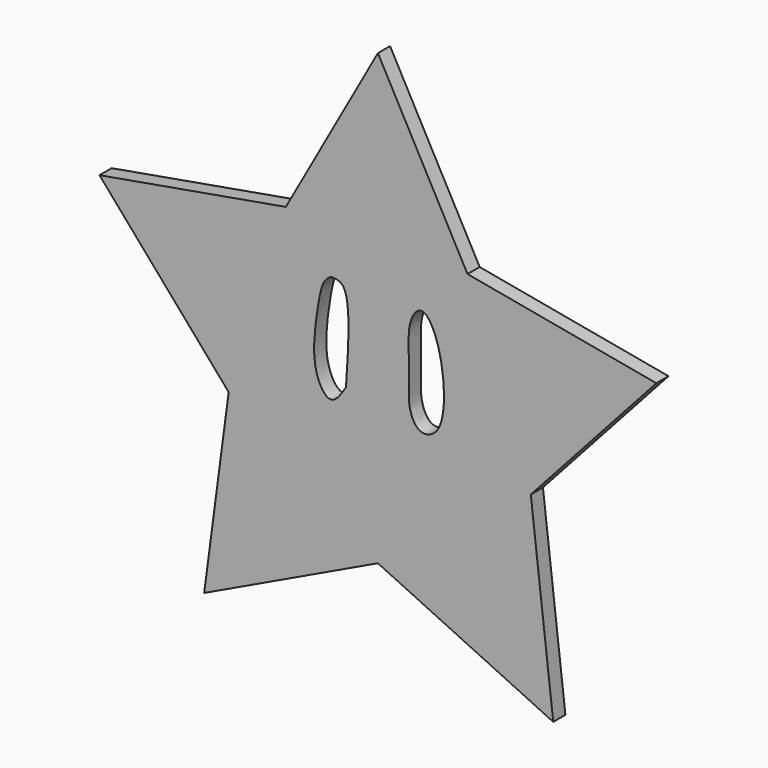
from build123d import *

# Parameters (mm, degrees)
F1_DEPTH = 2
F3_DEPTH = 25


with BuildPart() as f1:
    # F0 (on Front) → F1 (new body)
    with BuildSketch(Plane.XZ):
        Polygon((-48.7309247255, 48.1939427555), (-73.2373036639, 43.8981056213), (-56.2486425042, 24.2983382195), (-59.4705231488, 0), (-36.618651832, 10.8738420531), (-13.5587416589, 0), (-16.5121313184, 25.3722984344), (0, 43.6296164989), (-24.835318327, 48.1939427555), (-36.618651832, 69.941624999), align=None)
    extrude(amount=F1_DEPTH)

    # F2 (on face) → F3 (cut)
    with BuildSketch(Plane.XZ.offset(2)):
        with BuildLine():
            add(Edge.make_bspline(
                [(-42.8241454065, 42.018674314), (-42.215811031, 42.0156652147), (-40.0248783805, 42.0048278626), (-40.4838324873, 34.9711646084), (-40.8153533936, 29.8904683441)],
                knots=[0, 0, 0, 0, 0.2776600072, 1, 1, 1, 1], degree=3))
            add(Edge.make_bspline(
                [(-42.8241454065, 42.018674314), (-43.1211611971, 41.817411735), (-43.9730260473, 41.2401746918), (-44.7285981197, 37.046533313), (-45.4586501607, 30.6342959102), (-42.8138464069, 26.7380268066), (-41.4719755399, 28.85470644), (-40.8153533936, 29.8904683441)],
                knots=[0, 0, 0, 0, 0.1173333317, 0.3365213034, 0.622595536, 0.815323415, 1, 1, 1, 1], degree=3))
        make_face()
        with BuildLine():
            add(Edge.make_bspline(
                [(-30.4665230215, 41.817411735), (-30.7828157907, 42.0132867548), (-31.5566720158, 42.0016665583), (-32.758418401, 39.7526667198), (-32.4605723261, 35.8588497009), (-32.5698270564, 31.5889371812), (-32.4797926297, 29.976349033), (-31.378124697, 27.4296174444), (-27.4746603802, 28.3933105876), (-27.939027342, 38.0017634716), (-29.776947659, 41.3903688148), (-30.4665230215, 41.817411735)],
                knots=[0, 0, 0, 0, 0.0595652349, 0.1516653863, 0.2790521251, 0.4073989231, 0.4888413673, 0.5825769232, 0.6810659238, 0.8701370299, 1, 1, 1, 1], degree=3))
        make_face()
    extrude(amount=-F3_DEPTH, mode=Mode.SUBTRACT)


solid = f1.part
